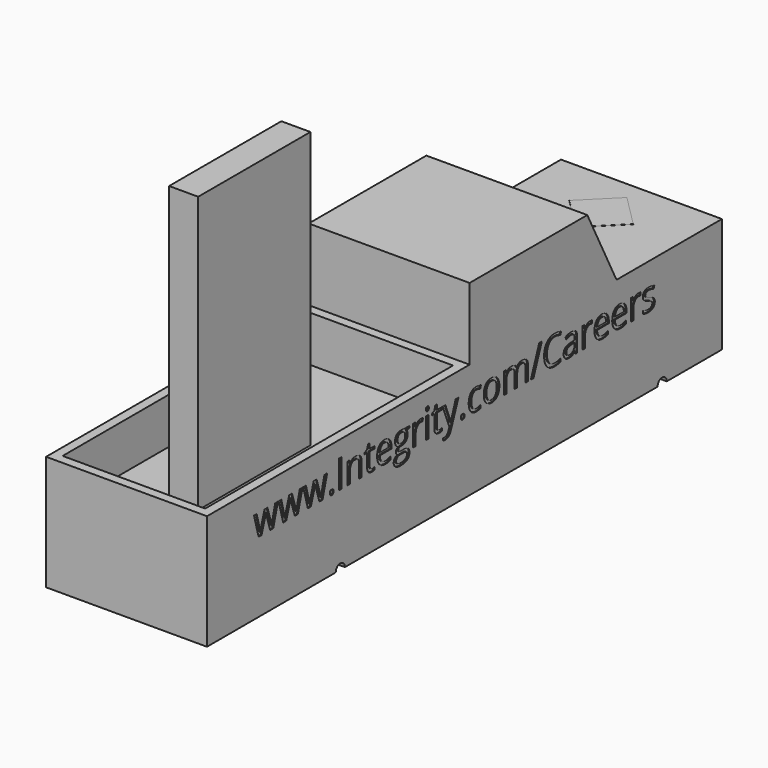
from build123d import *

# Parameters (mm, degrees)
F0_W         = 44.45
F0_H         = 31.75
F1_DEPTH     = 177.8
F3_DEPTH     = 44.451
F4_W         = 39.37
F4_H         = 85.598
F5_DEPTH     = 12.7
F7_DEPTH     = 0.0508
F8_TEXT_SIZE = 10.9310624086
F9_DEPTH     = 0.254
F10_W        = 8.029172197
F10_H        = 38.760477677
F11_DEPTH    = 76.2
F13_DEPTH    = 22.225


# Not quite as in the source:
# - Text() gives the source's letters only with a copy of the font that has no kerning and outlines rounded to 1/6400 em; it was checked with that copy


with BuildPart() as f1:
    # F0 (on Front) → F1 (new body)
    with BuildSketch(Plane.XZ):
        Rectangle(F0_W, F0_H)
    extrude(amount=-F1_DEPTH)

    # F2 (on face) → F3 (cut, through all)
    with BuildSketch(Plane.YZ.offset(22.225)):
        with BuildLine():
            ThreePointArc((47.625, -15.875), (46.0375, -14.2875), (44.45, -15.875))
            Line((44.45, -15.875), (47.625, -15.875))
        make_face()
        with BuildLine():
            ThreePointArc((158.75, -15.875), (157.1625, -14.2875), (155.575, -15.875))
            Line((155.575, -15.875), (158.75, -15.875))
        make_face()
    extrude(amount=-F3_DEPTH, mode=Mode.SUBTRACT)

    # F4 (on face) → F5 (cut)
    with BuildSketch(Plane.XY.offset(15.875)):
        with Locations((0, 45.339)):
            Rectangle(F4_W, F4_H)
    extrude(amount=-F5_DEPTH, mode=Mode.SUBTRACT)

    # F6 (on face) → F7 (join)
    with BuildSketch(Plane.XY.offset(15.875)):
        Polygon((8.8464077562, 163.9133337885), (0, 172.7597415447), (-8.8464077562, 163.9133337885), (0, 155.0669260323), align=None)
    extrude(amount=F7_DEPTH)

    # F8 (on face) → F9 (cut)
    with BuildSketch(Plane.YZ.offset(22.225)):
        with Locations((16.0976015031, 3.6293484736)):
            Text('www.Integrity.com/Careers', F8_TEXT_SIZE, font='Open Sans', text_align=(TextAlign.LEFT, TextAlign.BOTTOM))
    extrude(amount=-F9_DEPTH, mode=Mode.SUBTRACT)

    # F10 (on face) → F11 (join)
    with BuildSketch(Plane.XY.offset(3.175)):
        with Locations((-0.3001601435, 39.4675349817)):
            Rectangle(F10_W, F10_H)
    extrude(amount=F11_DEPTH)

    # F12 (on Right) → F13 (join, symmetric)
    with BuildSketch(Plane.YZ):
        Polygon((90.678, 15.875), (141.4068940412, 15.875), (131.3073236723, 35.7410460711), (90.678, 35.7410460711), align=None)
    extrude(amount=F13_DEPTH, both=True)


solid = f1.part
